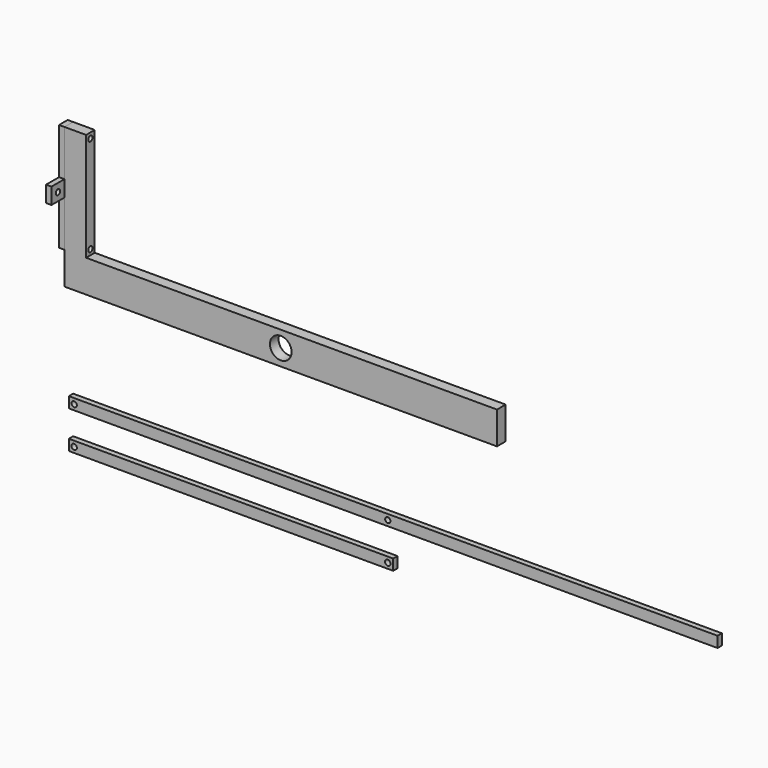
from build123d import *

# Parameters (mm, degrees)
F0_W     = 25.4
F0_H     = 127
F0_H_2   = 38.1
F0_W_2   = 482.6
F0_R     = 12.7
F1_DEPTH = 12.7
F2_R     = 3.175
F3_DEPTH = 25.4
F2_W     = 12.7
F2_H     = 53.975
F2_H_2   = 19.05
F2_W_2   = 19.05
F4_DEPTH = 6.35
F0_W_3   = 762
F0_H_3   = 12.7
F0_R_2   = 3.1045805256
F5_DEPTH = 6.35
F0_W_4   = 381
F0_R_3   = 3.175


with BuildPart() as f1:
    # F0 (on Front) → F1 (new body)
    with BuildSketch(Plane.XZ):
        with Locations((12.7, 63.5)):
            Rectangle(F0_W, F0_H)
        with Locations((12.7, -19.05)):
            Rectangle(F0_W, F0_H_2)
        with Locations((266.7, -19.05)):
            Rectangle(F0_W_2, F0_H_2)
        with Locations((254, -19.05)):
            Circle(F0_R, mode=Mode.SUBTRACT)
    extrude(amount=F1_DEPTH)

    # F2 (on face) → F3 (cut)
    with BuildSketch(Plane(origin=(0, 0, 0), x_dir=(0, -1, 0), z_dir=(-1, 0, 0))):
        with Locations((6.35, 120.65)):
            Circle(F2_R)
        with Locations((6.35, 6.35)):
            Circle(F2_R)
    extrude(amount=-F3_DEPTH, mode=Mode.SUBTRACT)


with BuildPart() as f4:
    # F2 (on face) → F4 (new body)
    with BuildSketch(Plane(origin=(0, 0, 0), x_dir=(0, -1, 0), z_dir=(-1, 0, 0))):
        with Locations((6.35, 100.0125)):
            Rectangle(F2_W, F2_H)
        with Locations((6.35, 120.65)):
            Circle(F2_R, mode=Mode.SUBTRACT)
        with Locations((6.35, 63.5)):
            Rectangle(F2_W, F2_H_2)
        with Locations((-9.525, 63.5)):
            Rectangle(F2_W_2, F2_H_2)
        with Locations((-9.525, 63.5)):
            Circle(F2_R, mode=Mode.SUBTRACT)
        with Locations((22.225, 63.5)):
            Rectangle(F2_W_2, F2_H_2)
        with Locations((22.225, 63.5)):
            Circle(F2_R, mode=Mode.SUBTRACT)
        with Locations((6.35, 26.9875)):
            Rectangle(F2_W, F2_H)
        with Locations((6.35, 6.35)):
            Circle(F2_R, mode=Mode.SUBTRACT)
    extrude(amount=F4_DEPTH)


with BuildPart() as f5:
    # F0 (on Front) → F5 (new body)
    with BuildSketch(Plane.XZ):
        with Locations((381, -160.2233456612)):
            Rectangle(F0_W_3, F0_H_3)
        with Locations((6.35, -160.2233456612)):
            Circle(F0_R_2, mode=Mode.SUBTRACT)
        with Locations((374.65, -160.2233456612)):
            Circle(F0_R_2, mode=Mode.SUBTRACT)
    extrude(amount=F5_DEPTH)


with BuildPart() as f5b:
    # F0 (on Front) → F5, piece 2 (new body)
    with BuildSketch(Plane.XZ):
        with Locations((190.5, -204.2886721134)):
            Rectangle(F0_W_4, F0_H_3)
        with Locations((6.35, -204.2886721134)):
            Circle(F0_R_3, mode=Mode.SUBTRACT)
        with Locations((374.65, -204.2886721134)):
            Circle(F0_R_3, mode=Mode.SUBTRACT)
    extrude(amount=F5_DEPTH)


solid = Compound([f1.part, f4.part, f5.part, f5b.part])
